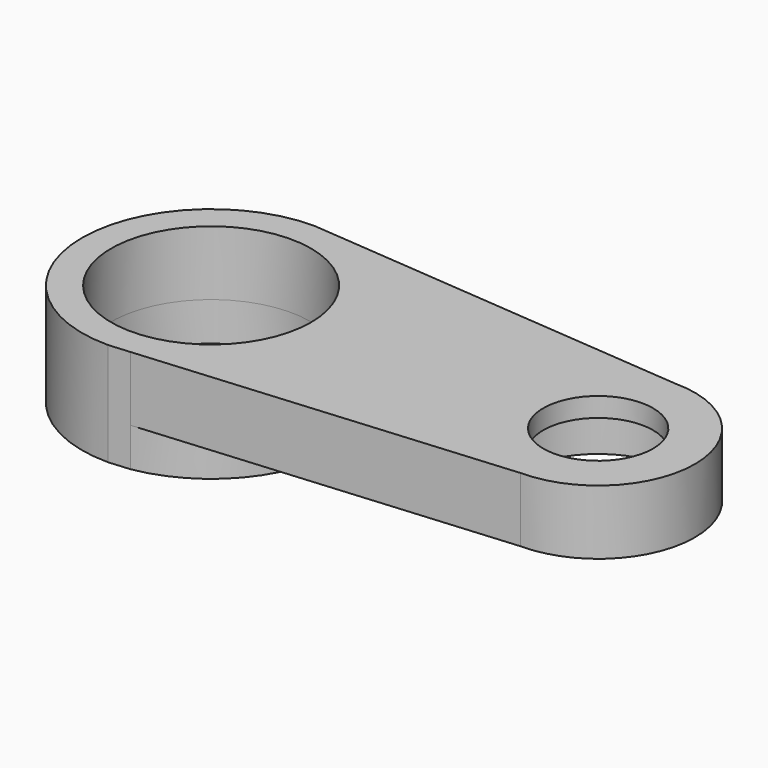
from build123d import *

# Parameters (mm, degrees)
F0_R     = 7.75
F0_R_2   = 6.25
F0_R_3   = 4.25
F1_DEPTH = 5
F2_DEPTH = 3
F3_DEPTH = 3.5


with BuildPart() as f1:
    # F0 (on Top) → F1 (new body)
    with BuildSketch(Plane.XY):
        with BuildLine():
            Line((1.6551724138, 9.8620689655), (0, 10))
            ThreePointArc((0, 10), (-10, 0), (0, -10))
            Line((0, -10), (1.6551724138, -9.8620689655))
            ThreePointArc((1.6551724138, -9.8620689655), (7.6338628537, -6.4594224147), (10, 0))
            ThreePointArc((10, 0), (7.6338628537, 6.4594224147), (1.6551724138, 9.8620689655))
        make_face()
        Circle(F0_R, mode=Mode.SUBTRACT)
        with BuildLine():
            Line((30, 7.5), (1.6551724138, 9.8620689655))
            ThreePointArc((1.6551724138, 9.8620689655), (7.6338628537, 6.4594224147), (10, 0))
            ThreePointArc((10, 0), (7.6338628537, -6.4594224147), (1.6551724138, -9.8620689655))
            Line((1.6551724138, -9.8620689655), (30, -7.5))
            ThreePointArc((30, -7.5), (22.5, 0), (30, 7.5))
        make_face()
        with BuildLine():
            ThreePointArc((37.5, 0), (35.3033008589, 5.3033008589), (30, 7.5))
            ThreePointArc((30, 7.5), (22.5, 0), (30, -7.5))
            ThreePointArc((30, -7.5), (35.3033008589, -5.3033008589), (37.5, 0))
        make_face()
        with Locations((30, 0)):
            Circle(F0_R_2, mode=Mode.SUBTRACT)
        with Locations((30, 0)):
            Circle(F0_R_2)
        with Locations((30, 0)):
            Circle(F0_R_3, mode=Mode.SUBTRACT)
    extrude(amount=F1_DEPTH)

    # F0 (on Top) → F2 (join)
    with BuildSketch(Plane.XY):
        with BuildLine():
            Line((1.6551724138, 9.8620689655), (0, 10))
            ThreePointArc((0, 10), (-10, 0), (0, -10))
            Line((0, -10), (1.6551724138, -9.8620689655))
            ThreePointArc((1.6551724138, -9.8620689655), (7.6338628537, -6.4594224147), (10, 0))
            ThreePointArc((10, 0), (7.6338628537, 6.4594224147), (1.6551724138, 9.8620689655))
        make_face()
        Circle(F0_R, mode=Mode.SUBTRACT)
    extrude(amount=-F2_DEPTH)

    # F0 (on Top) → F3 (cut)
    with BuildSketch(Plane.XY):
        with Locations((30, 0)):
            Circle(F0_R_2)
        with Locations((30, 0)):
            Circle(F0_R_3, mode=Mode.SUBTRACT)
    extrude(amount=F3_DEPTH, mode=Mode.SUBTRACT)


solid = f1.part
